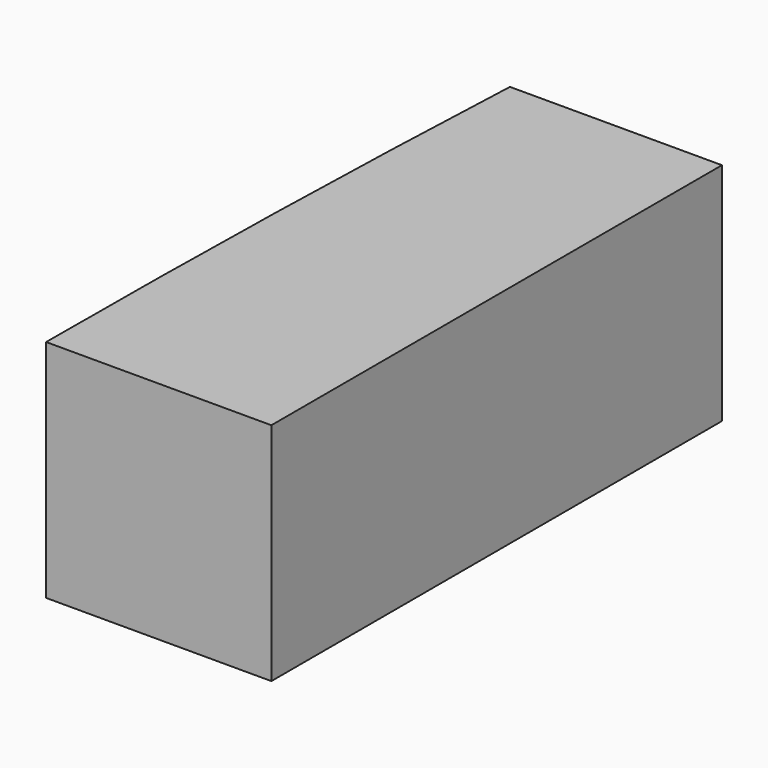
from build123d import *

# Parameters (mm, degrees)
F1_DEPTH = 4


with BuildPart() as f1:
    # F0 (on Top) → F1 (new body)
    with BuildSketch(Plane.XY):
        with BuildLine():
            Line((-207.9103297946, 10), (-211.6742494345, 10))
            ThreePointArc((-211.6742494345, 10), (-211.8513014833, 5.0013931543), (-211.9103297946, 0))
            Line((-211.9103297946, 0), (-207.9103297946, 0))
            Line((-207.9103297946, 0), (-207.9103297946, 10))
        make_face()
    extrude(amount=F1_DEPTH)


solid = f1.part
